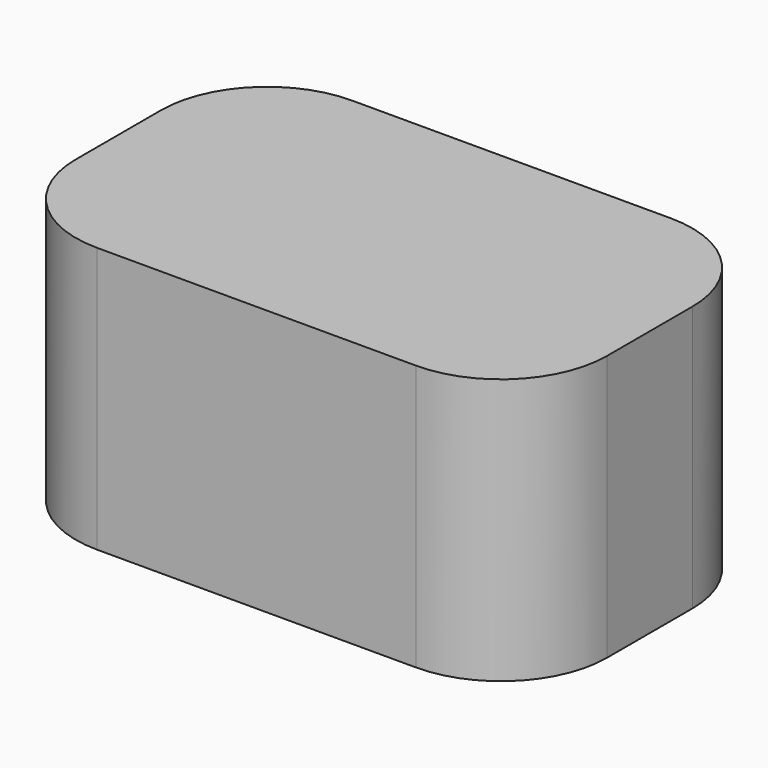
from build123d import *

# Parameters (mm, degrees)
F0_W     = 50
F0_H     = 30
F1_DEPTH = 25
F2_R     = 10


# Not quite as in the source:
# - a feature of the source that left no trace in its solid (it failed there, or was rolled back) is left out


with BuildPart() as f1:
    # F0 (on Top) → F1 (new body)
    with BuildSketch(Plane.XY):
        Rectangle(F0_W, F0_H)
    extrude(amount=F1_DEPTH)

    # F2
    f2_edges = [f1.edges().sort_by_distance(p)[0] for p in [
        (25, -15, 12.5),
        (-25, -15, 12.5),
        (25, 15, 12.5),
        (-25, 15, 12.5),
    ]]
    fillet(f2_edges, radius=F2_R)


solid = f1.part
